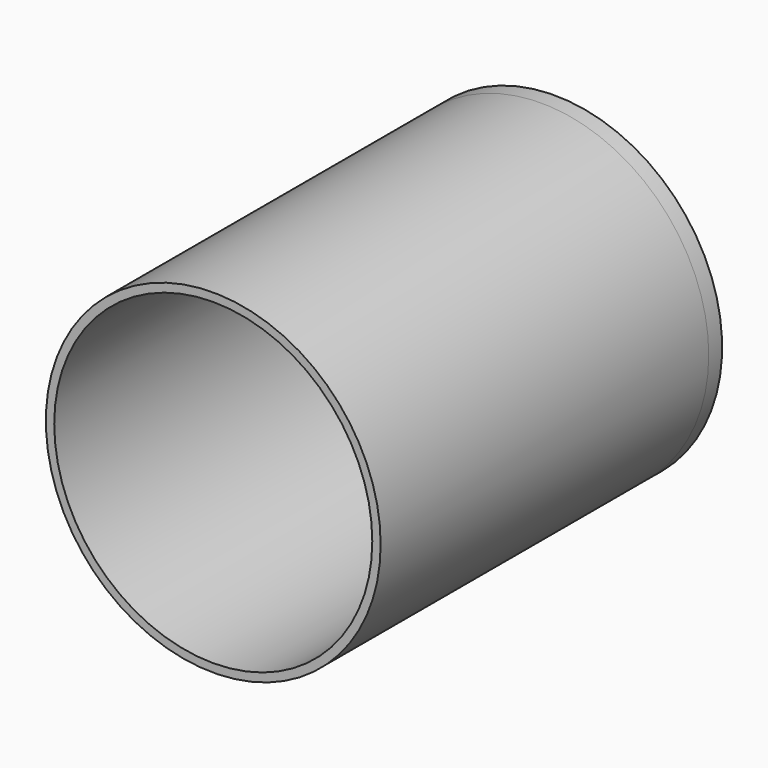
from build123d import *

# Parameters (mm, degrees)
F0_R     = 20
F0_R_2   = 19
F1_DEPTH = 22
F2_R     = 20
F2_R_2   = 19
F3_DEPTH = 27
F4_R     = 20
F4_R_2   = 19
F5_DEPTH = 2


with BuildPart() as f1:
    # F0 (on Front) → F1 (new body)
    with BuildSketch(Plane.XZ):
        Circle(F0_R)
        Circle(F0_R_2, mode=Mode.SUBTRACT)
    extrude(amount=F1_DEPTH)

    # F2 (on face) → F3 (join)
    with BuildSketch(Plane.XZ.offset(22)):
        Circle(F2_R)
        Circle(F2_R_2, mode=Mode.SUBTRACT)
    extrude(amount=F3_DEPTH)

    # F4 (on face) → F5 (join)
    with BuildSketch(Plane(origin=(0, 0, 0), x_dir=(-1, 0, 0), z_dir=(0, 1, 0))):
        Circle(F4_R)
        Circle(F4_R_2, mode=Mode.SUBTRACT)
        Circle(F4_R_2)
    extrude(amount=F5_DEPTH)


solid = f1.part
